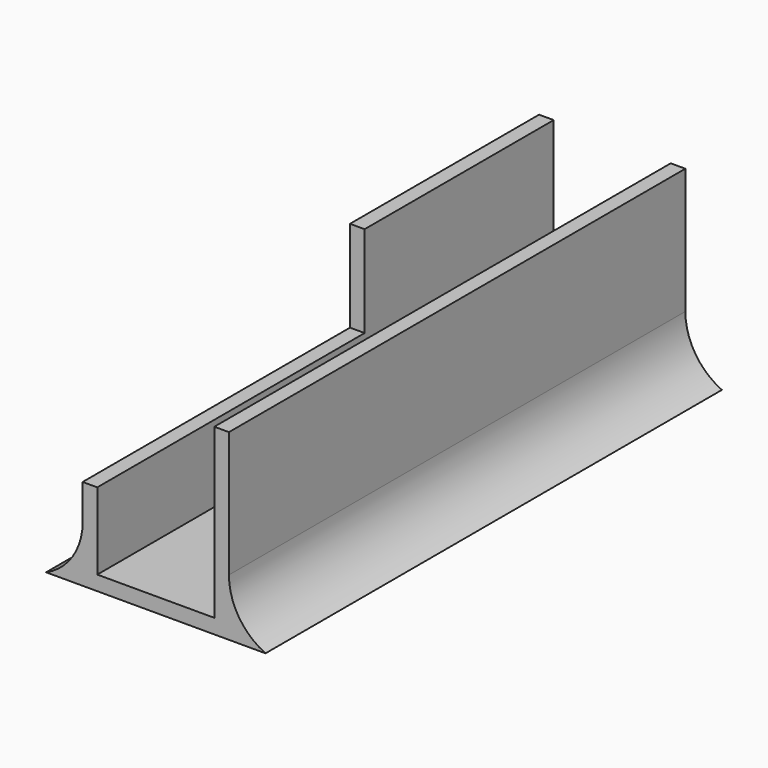
from build123d import *

# Parameters (mm, degrees)
F0_W     = 2
F0_H     = 78
F1_DEPTH = 25
F0_W_2   = 16
F2_DEPTH = 2
F3_W     = 45.6874087788
F3_H     = 12.5
F4_DEPTH = 10
F7_DEPTH = 78
F8_DEPTH = 78


# Not quite as in the source:
# - a feature names something its author has since deleted; it is built from what else it names


with BuildPart() as f1:
    # F0 (on Top) → F1 (new body)
    with BuildSketch(Plane.XY):
        with Locations((9, 0)):
            Rectangle(F0_W, F0_H)
    extrude(amount=F1_DEPTH)



with BuildPart() as f1b:
    # F0 (on Top) → F1, piece 2 (new body)
    with BuildSketch(Plane.XY):
        with Locations((-9, 0)):
            Rectangle(F0_W, F0_H)
    extrude(amount=F1_DEPTH)


with BuildPart() as f1_1:
    add(f1.part)

    add(f1b.part)  # F2 merges F1b
    # F0 (on Top) → F2 (join)
    with BuildSketch(Plane.XY):
        with Locations((9, 0)):
            Rectangle(F0_W, F0_H)
        Rectangle(F0_W_2, F0_H)
        with Locations((-9, 0)):
            Rectangle(F0_W, F0_H)
    extrude(amount=F2_DEPTH)

    # F3 (on face) → F4 (cut)
    with BuildSketch(Plane(origin=(-10, 0, 0), x_dir=(0, -1, 0), z_dir=(-1, 0, 0))):
        with Locations((16.1562956106, 18.75)):
            Rectangle(F3_W, F3_H)
    extrude(amount=-F4_DEPTH, mode=Mode.SUBTRACT)

    # F6 (on face) → F7 (join)
    with BuildSketch(Plane(origin=(0, 39, 0), x_dir=(-1, 0, 0), z_dir=(0, 1, 0))):
        with BuildLine():
            ThreePointArc((-10, 7.8135579824), (-11.356996059, 3.1753555196), (-15, 0))
            Line((-15, 0), (-10, 0))
            Line((-10, 0), (-10, 7.8135579824))
        make_face()
    extrude(amount=-F7_DEPTH)

    # F5 (on face) → F8 (join)
    with BuildSketch(Plane(origin=(0, 39, 0), x_dir=(-1, 0, 0), z_dir=(0, 1, 0))):
        with BuildLine():
            Line((10, 0), (15, 0))
            ThreePointArc((15, 0), (11.360255444, 3.0951443467), (10, 7.6752495952))
            Line((10, 7.6752495952), (10, 0))
        make_face()
    extrude(amount=-F8_DEPTH)


solid = f1_1.part
